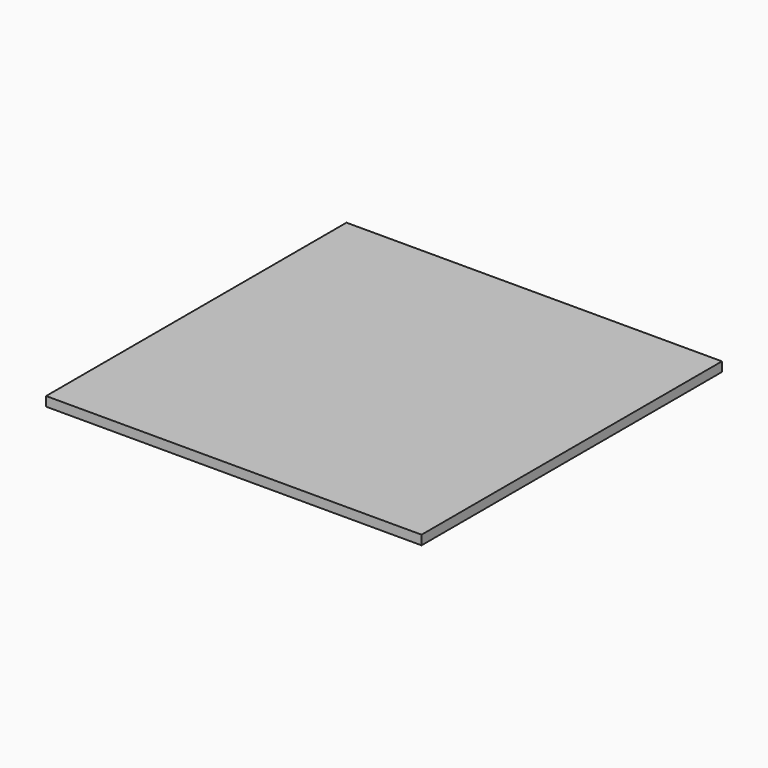
from build123d import *

# Parameters (mm, degrees)
F0_W     = 127
F0_H     = 127
F1_DEPTH = 3.175


# Not quite as in the source:
# - a length typed as a fraction of an inch, garbled in the dataset ("3 / 203.2 mm" for 3/8 in), is restored


with BuildPart() as f1:
    # F0 (on Top) → F1 (new body)
    with BuildSketch(Plane.XY):
        with Locations((-63.5, -63.5)):
            Rectangle(F0_W, F0_H)
    extrude(amount=F1_DEPTH)


solid = f1.part
